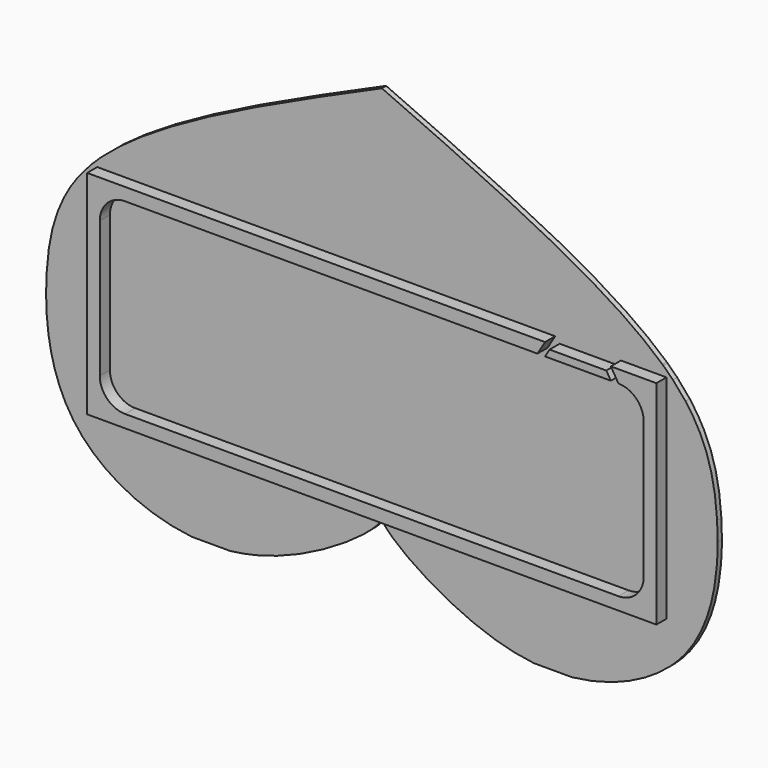
from build123d import *

# Parameters (mm, degrees)
F0_W     = 584.2
F0_H     = 219.71
F1_DEPTH = 5.334
F2_W     = 571.5
F2_H     = 213.36
F2_W_2   = 546.1
F2_H_2   = 187.96
F3_DEPTH = 12.7
F4_R     = 25.4
F6_DEPTH = 12.7
F7_W     = 12.7
F7_H     = 109.855
F8_DEPTH = 5.334


# Not quite as in the source:
# - a feature names something its author has since deleted; it is built from what else it names


with BuildPart() as f1:
    # F0 (on Front) → F1 (new body)
    with BuildSketch(Plane.XZ):
        with Locations((-292.1, 109.855)):
            Rectangle(F0_W, F0_H)
    extrude(amount=F1_DEPTH)

    # F2 (on face) → F3 (join)
    with BuildSketch(Plane.XZ.offset(5.334)):
        with Locations((-292.1, 113.03)):
            Rectangle(F2_W, F2_H)
        with Locations((-292.1, 113.03)):
            Rectangle(F2_W_2, F2_H_2, mode=Mode.SUBTRACT)
    extrude(amount=F3_DEPTH)

    # F4
    f4_edges = [f1.edges().sort_by_distance(p)[0] for p in [
        (-565.15, -11.684, 207.01),
        (-19.05, -11.684, 207.01),
        (-19.05, -11.684, 19.05),
        (-565.15, -11.684, 19.05),
    ]]
    fillet(f4_edges, radius=F4_R)

    # F5 (on face) → F6 (cut)
    with BuildSketch(Plane.XZ.offset(18.034)):
        Polygon((-118.11, 219.71), (-125.73, 207.01), (-118.11, 207.01), (-113.5820166854, 214.5566388576), (-110.49, 219.71), align=None)
        Polygon((-56.5979833146, 214.5566388576), (-52.07, 207.01), (-44.45, 207.01), (-52.07, 219.71), (-59.69, 219.71), align=None)
        Polygon((-59.69, 219.71), (-110.49, 219.71), (-113.5820166854, 214.5566388576), (-56.5979833146, 214.5566388576), align=None)
    extrude(amount=-F6_DEPTH, mode=Mode.SUBTRACT)

    # F7 (on face) → F8 (join)
    with BuildSketch(Plane(origin=(0, 0, 0), x_dir=(-1, 0, 0), z_dir=(0, 1, 0))):
        with BuildLine():
            Line((292.1, 0), (0, 0))
            Line((0, 0), (-12.7, 0))
            Line((-12.7, 0), (-12.7, -18.4187279276))
            Line((-12.7, -18.4187279276), (273.05, -18.4187279276))
            add(Edge.make_bspline(
                [(292.1, 0), (287.6007994264, -5.2493532032), (283.1015988528, -10.4987064064), (273.05, -18.4187279276)],
                knots=[0, 0, 0, 0, 0.0728769887, 0.0728769887, 0.0728769887, 0.0728769887], degree=3))
        make_face()
        with Locations((-6.35, 54.9275)):
            Rectangle(F7_W, F7_H)
        with BuildLine():
            Line((-12.7, -18.4187279276), (-12.7, 0))
            Line((-12.7, 0), (-12.7, 109.855))
            Line((-12.7, 109.855), (-44.45, 109.855))
            add(Edge.make_bspline(
                [(-45.0211916342, 91.2168765815), (-45.0211916609, 97.5162300277), (-44.815953395, 103.7471754572), (-44.45, 109.855)],
                knots=[0.5639304479, 0.5639304479, 0.5639304479, 0.5639304479, 0.5870347541, 0.5870347541, 0.5870347541, 0.5870347541], degree=3))
            add(Edge.make_bspline(
                [(-12.7, -18.4187279276), (-37.5240442459, 12.5724048939), (-45.0211914731, 53.1440785365), (-45.0211916342, 91.2168765815)],
                knots=[0.4242898339, 0.4242898339, 0.4242898339, 0.4242898339, 0.5639304479, 0.5639304479, 0.5639304479, 0.5639304479], degree=3))
        make_face()
        with BuildLine():
            Line((584.2, 0), (292.1, 0))
            add(Edge.make_bspline(
                [(292.1, 0), (296.5992005736, -5.2493532032), (301.0984011472, -10.4987064064), (311.15, -18.4187279276)],
                knots=[0, 0, 0, 0, 0.0728769887, 0.0728769887, 0.0728769887, 0.0728769887], degree=3))
            Line((311.15, -18.4187279276), (596.9, -18.4187279276))
            Line((596.9, -18.4187279276), (596.9, 0))
            Line((596.9, 0), (584.2, 0))
        make_face()
        with BuildLine():
            Line((-12.7, 109.855), (0, 109.855))
            Line((0, 109.855), (0, 219.71))
            add(Edge.make_bspline(
                [(-12.7, 204.8965850641), (-8.9139816017, 209.8723459181), (-4.696536047, 214.8060326557), (0, 219.71)],
                knots=[0.7188244338, 0.7188244338, 0.7188244338, 0.7188244338, 0.7411532433, 0.7411532433, 0.7411532433, 0.7411532433], degree=3))
            Line((-12.7, 204.8965850641), (-12.7, 109.855))
        make_face()
        with BuildLine():
            Line((-44.45, 109.855), (-12.7, 109.855))
            Line((-12.7, 109.855), (-12.7, 204.8965850641))
            add(Edge.make_bspline(
                [(-44.45, 109.855), (-42.3625587956, 144.6947495266), (-35.0459362357, 175.5285199707), (-12.7, 204.8965850641)],
                knots=[0.5870347541, 0.5870347541, 0.5870347541, 0.5870347541, 0.7188244338, 0.7188244338, 0.7188244338, 0.7188244338], degree=3))
        make_face()
        with BuildLine():
            Line((273.05, -18.4187279276), (-12.7, -18.4187279276))
            add(Edge.make_bspline(
                [(101.1778231225, -76.2), (55.3698473988, -71.3735043498), (12.4455878923, -49.8112861475), (-12.7, -18.4187279276)],
                knots=[0.2828404673, 0.2828404673, 0.2828404673, 0.2828404673, 0.4242898339, 0.4242898339, 0.4242898339, 0.4242898339], degree=3))
            Line((101.1778231225, -76.2), (139.7, -76.2))
            add(Edge.make_bspline(
                [(273.05, -18.4187279276), (249.5100545477, -36.9667099273), (195.5177305995, -70.1620926298), (139.7, -76.2)],
                knots=[0.0728769887, 0.0728769887, 0.0728769887, 0.0728769887, 0.2435483779, 0.2435483779, 0.2435483779, 0.2435483779], degree=3))
        make_face()
        with BuildLine():
            Line((596.9, -18.4187279276), (311.15, -18.4187279276))
            add(Edge.make_bspline(
                [(311.15, -18.4187279276), (334.6899454523, -36.9667099273), (388.6822694005, -70.1620926298), (444.5, -76.2)],
                knots=[0.0728769887, 0.0728769887, 0.0728769887, 0.0728769887, 0.2435483779, 0.2435483779, 0.2435483779, 0.2435483779], degree=3))
            Line((444.5, -76.2), (483.0221768775, -76.2))
            add(Edge.make_bspline(
                [(483.0221768775, -76.2), (528.8301526012, -71.3735043498), (571.7544121077, -49.8112861475), (596.9, -18.4187279276)],
                knots=[0.2828404673, 0.2828404673, 0.2828404673, 0.2828404673, 0.4242898339, 0.4242898339, 0.4242898339, 0.4242898339], degree=3))
        make_face()
        with Locations((590.55, 54.9275)):
            Rectangle(F7_W, F7_H)
        with BuildLine():
            add(Edge.make_bspline(
                [(0, 219.71), (3.0172855437, 222.8605496023), (6.2323113272, 225.9988327955), (9.6341187106, 229.1255293763)],
                knots=[0.7411532433, 0.7411532433, 0.7411532433, 0.7411532433, 0.7554983677, 0.7554983677, 0.7554983677, 0.7554983677], degree=3))
            Line((0, 219.71), (292.1, 219.71))
            Line((292.1, 219.71), (9.6341187106, 229.1255293763))
        make_face()
        with BuildLine():
            Line((596.9, 0), (596.9, -18.4187279276))
            add(Edge.make_bspline(
                [(596.9, -18.4187279276), (621.7240438178, 12.5724043593), (629.2211912145, 53.144077137), (629.2211916342, 91.2168746116)],
                knots=[0.4242898339, 0.4242898339, 0.4242898339, 0.4242898339, 0.5639304455, 0.5639304455, 0.5639304455, 0.5639304455], degree=3))
            add(Edge.make_bspline(
                [(629.2211916342, 91.2168746116), (629.2211917037, 97.5162287286), (629.0159534331, 103.7471748205), (628.65, 109.855)],
                knots=[0.5639304455, 0.5639304455, 0.5639304455, 0.5639304455, 0.5870347541, 0.5870347541, 0.5870347541, 0.5870347541], degree=3))
            Line((628.65, 109.855), (596.9, 109.855))
            Line((596.9, 109.855), (596.9, 0))
        make_face()
        with BuildLine():
            Line((584.2, 219.71), (584.2, 109.855))
            Line((584.2, 109.855), (596.9, 109.855))
            Line((596.9, 109.855), (596.9, 204.8965850641))
            add(Edge.make_bspline(
                [(596.9, 204.8965850641), (593.1139816017, 209.8723459181), (588.896536047, 214.8060326557), (584.2, 219.71)],
                knots=[0.7188244338, 0.7188244338, 0.7188244338, 0.7188244338, 0.7411532433, 0.7411532433, 0.7411532433, 0.7411532433], degree=3))
        make_face()
        with BuildLine():
            add(Edge.make_bspline(
                [(9.6341187106, 229.1255293763), (9.9041896656, 229.3737591661), (10.1754378752, 229.6219159272), (10.4478578559, 229.87)],
                knots=[0.7554983677, 0.7554983677, 0.7554983677, 0.7554983677, 0.7566372333, 0.7566372333, 0.7566372333, 0.7566372333], degree=3))
            Line((9.6341187106, 229.1255293763), (292.1, 219.71))
            Line((292.1, 219.71), (574.5658812894, 229.1255293763))
            add(Edge.make_bspline(
                [(574.5658812894, 229.1255293763), (574.2958103344, 229.3737591661), (574.0245621248, 229.6219159272), (573.7521421441, 229.87)],
                knots=[0.7554983677, 0.7554983677, 0.7554983677, 0.7554983677, 0.7566372333, 0.7566372333, 0.7566372333, 0.7566372333], degree=3))
            Line((573.7521421441, 229.87), (514.35, 229.87))
            Line((514.35, 229.87), (292.1, 229.87))
            Line((292.1, 229.87), (69.85, 229.87))
            Line((69.85, 229.87), (10.4478578559, 229.87))
        make_face()
        with BuildLine():
            Line((574.5658812894, 229.1255293763), (292.1, 219.71))
            Line((292.1, 219.71), (584.2, 219.71))
            add(Edge.make_bspline(
                [(584.2, 219.71), (581.1827144563, 222.8605496023), (577.9676886728, 225.9988327955), (574.5658812894, 229.1255293763)],
                knots=[0.7411532433, 0.7411532433, 0.7411532433, 0.7411532433, 0.7554983677, 0.7554983677, 0.7554983677, 0.7554983677], degree=3))
        make_face()
        with BuildLine():
            Line((596.9, 204.8965850641), (596.9, 109.855))
            Line((596.9, 109.855), (628.65, 109.855))
            add(Edge.make_bspline(
                [(628.65, 109.855), (626.5625587956, 144.6947495266), (619.2459362357, 175.5285199707), (596.9, 204.8965850641)],
                knots=[0.5870347541, 0.5870347541, 0.5870347541, 0.5870347541, 0.7188244338, 0.7188244338, 0.7188244338, 0.7188244338], degree=3))
        make_face()
        with BuildLine():
            add(Edge.make_bspline(
                [(10.4478578559, 229.87), (68.6609423687, 282.8827748158), (180.3804711844, 332.5763874079), (292.1, 382.27)],
                knots=[0.7566372333, 0.7566372333, 0.7566372333, 0.7566372333, 1, 1, 1, 1], degree=3))
            Line((10.4478578559, 229.87), (69.85, 229.87))
            Line((69.85, 229.87), (292.1, 229.87))
            Line((292.1, 229.87), (292.1, 382.27))
        make_face()
        with BuildLine():
            add(Edge.make_bspline(
                [(573.7521421441, 229.87), (515.5390576313, 282.8827748158), (403.8195288156, 332.5763874079), (292.1, 382.27)],
                knots=[0.7566372333, 0.7566372333, 0.7566372333, 0.7566372333, 1, 1, 1, 1], degree=3))
            Line((292.1, 382.27), (292.1, 229.87))
            Line((292.1, 229.87), (514.35, 229.87))
            Line((514.35, 229.87), (573.7521421441, 229.87))
        make_face()
    extrude(amount=-F8_DEPTH)


solid = f1.part
